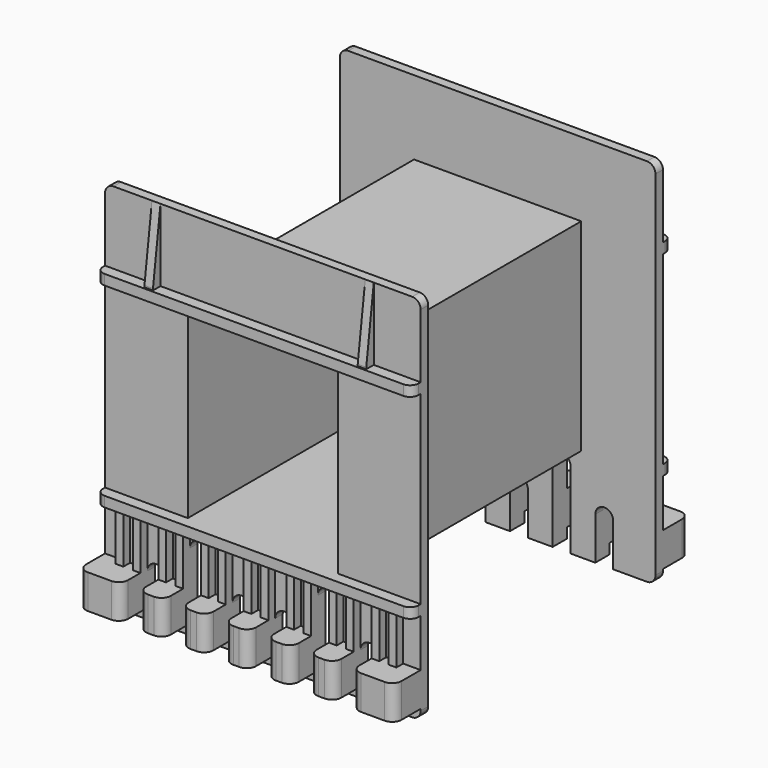
from build123d import *

# Parameters (mm, degrees)
F2_START  = 16.65
F1_W      = 37
F1_H      = 43.4
F1_W_2    = 17.6
F1_H_2    = 21.7
F2_DEPTH  = 1.1
F3_W      = 37
F3_H      = 1.2
F4_DEPTH  = 1.3
F6_DEPTH  = 1.3
F7_W      = 1
F7_H      = 8.5
F9_DEPTH  = 1.1
F8_W      = 1
F8_H      = 8.5
F10_DEPTH = 1.1
F11_SIZE2 = 8.3
F11_SIZE  = 1.1
F12_W     = 0.9
F12_H     = 10.8
F13_DEPTH = 1
F14_W     = 2.05
F14_H     = 4
F14_W_2   = 0.9
F14_W_3   = 1.1
F14_H_2   = 3.9999026618
F15_DEPTH = 3.9
F16_W     = 2.1
F16_H     = 5
F17_W     = 2.1
F17_H     = 9
F18_W     = 2.1
F18_H     = 5
F19_W     = 2.1
F19_H     = 5
F20_W     = 2.1
F20_H     = 9
F21_W     = 2.1
F21_H     = 5
F22_DEPTH = 2.5
F23_R     = 1
F24_R     = 1.1
F27_W     = 19.6
F27_H     = 23.7
F27_W_2   = 17.6
F27_H_2   = 21.7
F28_DEPTH = 17.5
F29_W     = 37.0475144535
F29_H     = 1.2455911213
F30_DEPTH = 2


with BuildPart() as f2:
    # F1 (on face) → F2 (new body)
    with BuildSketch(Plane.XZ.offset(F2_START)):
        with Locations((0, 21.6187323556)):
            Rectangle(F1_W, F1_H)
        with Locations((0, 22.7687323556)):
            Rectangle(F1_W_2, F1_H_2, mode=Mode.SUBTRACT)
    extrude(amount=F2_DEPTH)

    # F3 (on face) → F4 (join)
    with BuildSketch(Plane.XZ.offset(17.75)):
        with Locations((0, 34.2187323556)):
            Rectangle(F3_W, F3_H)
    extrude(amount=F4_DEPTH)

    # F5 (on face) → F6 (join)
    with BuildSketch(Plane.XZ.offset(17.75)):
        Polygon((-18.5, 11.9187323556), (-18.5, 10.7187323556), (18.5, 10.7187323556), (18.5, 11.9187323556), (8.8, 11.9187323556), (-8.8, 11.9187323556), align=None)
    extrude(amount=F6_DEPTH)

    # F7 (on face) → F9 (join)
    with BuildSketch(Plane.XZ.offset(17.75)):
        with Locations((-12.5, 39.0687323556)):
            Rectangle(F7_W, F7_H)
    extrude(amount=F9_DEPTH)

    # F8 (on face) → F10 (join)
    with BuildSketch(Plane.XZ.offset(17.75)):
        with Locations((12.5, 39.0687323556)):
            Rectangle(F8_W, F8_H)
    extrude(amount=F10_DEPTH)

    # F11
    f11_edges = [f2.edges().sort_by_distance(p)[0] for p in [
        (-12.5, -18.85, 43.318732),
        (12.5, -18.85, 43.318732),
    ]]
    f11_side = f2.faces().sort_by_distance((0, -17.25641, 43.318732))[0]
    chamfer(f11_edges, length=F11_SIZE, length2=F11_SIZE2, reference=f11_side)

    # F12 (on face) → F13 (join)
    with BuildSketch(Plane.XZ.offset(17.75)):
        with Locations((-16, 5.3187323556)):
            Rectangle(F12_W, F12_H)
        with Locations((-14, 5.3187323556)):
            Rectangle(F12_W, F12_H)
        with Locations((-11, 5.3187323556)):
            Rectangle(F12_W, F12_H)
        with Locations((-9, 5.3187323556)):
            Rectangle(F12_W, F12_H)
        with Locations((-6, 5.3187323556)):
            Rectangle(F12_W, F12_H)
        with Locations((-4, 5.3187323556)):
            Rectangle(F12_W, F12_H)
        with Locations((-1, 5.3187323556)):
            Rectangle(F12_W, F12_H)
        with Locations((1, 5.3187323556)):
            Rectangle(F12_W, F12_H)
        with Locations((4, 5.3187323556)):
            Rectangle(F12_W, F12_H)
        with Locations((6, 5.3187323556)):
            Rectangle(F12_W, F12_H)
        with Locations((9, 5.3187323556)):
            Rectangle(F12_W, F12_H)
        with Locations((11, 5.3187323556)):
            Rectangle(F12_W, F12_H)
        with Locations((14, 5.3187323556)):
            Rectangle(F12_W, F12_H)
        with Locations((16, 5.3187323556)):
            Rectangle(F12_W, F12_H)
    extrude(amount=F13_DEPTH)

    # F14 (on face) → F15 (join)
    with BuildSketch(Plane.XZ.offset(17.75)):
        with Locations((-17.475, 3.1187323556)):
            Rectangle(F14_W, F14_H)
        with Locations((-16, 3.1187323556)):
            Rectangle(F14_W_2, F14_H)
        with Locations((-15, 3.1187323556)):
            Rectangle(F14_W_3, F14_H)
        with Locations((-14, 3.1187323556)):
            Rectangle(F14_W_2, F14_H)
        with Locations((-11, 3.1186836865)):
            Rectangle(F14_W_2, F14_H_2)
        with Locations((-10, 3.1186836865)):
            Rectangle(F14_W_3, F14_H_2)
        with Locations((-9, 3.1186836865)):
            Rectangle(F14_W_2, F14_H_2)
        with Locations((-6, 3.1186836865)):
            Rectangle(F14_W_2, F14_H_2)
        with Locations((-5, 3.1186836865)):
            Rectangle(F14_W_3, F14_H_2)
        with Locations((-4, 3.1186836865)):
            Rectangle(F14_W_2, F14_H_2)
        with Locations((-1, 3.1187323556)):
            Rectangle(F14_W_2, F14_H)
        with Locations((0, 3.1187323556)):
            Rectangle(F14_W_3, F14_H)
        with Locations((1, 3.1187323556)):
            Rectangle(F14_W_2, F14_H)
        with Locations((4, 3.1187323556)):
            Rectangle(F14_W_2, F14_H)
        with Locations((5, 3.1187323556)):
            Rectangle(F14_W_3, F14_H)
        with Locations((6, 3.1187323556)):
            Rectangle(F14_W_2, F14_H)
        with Locations((9, 3.1187323556)):
            Rectangle(F14_W_2, F14_H)
        with Locations((10, 3.1187323556)):
            Rectangle(F14_W_3, F14_H)
        with Locations((11, 3.1187323556)):
            Rectangle(F14_W_2, F14_H)
        with Locations((14, 3.1187323556)):
            Rectangle(F14_W_2, F14_H)
        with Locations((15, 3.1187323556)):
            Rectangle(F14_W_3, F14_H)
        with Locations((16, 3.1187323556)):
            Rectangle(F14_W_2, F14_H)
        with Locations((17.475, 3.1187323556)):
            Rectangle(F14_W, F14_H)
    extrude(amount=F15_DEPTH)

    # F16 (on face) + F17 (on face) + F18 (on face) + F19 (on face) + F20 (on face) + F21 (on face) → F22 (cut, symmetric)
    with BuildSketch(Plane.XZ.offset(17.75)):
        with Locations((-12.5, 2.4187323556)):
            Rectangle(F16_W, F16_H)
        with BuildLine():
            ThreePointArc((-11.45, 4.9187323556), (-12.5, 5.9687323556), (-13.55, 4.9187323556))
            Line((-13.55, 4.9187323556), (-11.45, 4.9187323556))
        make_face()
    with BuildSketch(Plane.XZ.offset(17.75)):
        with Locations((-7.5, 4.4187323556)):
            Rectangle(F17_W, F17_H)
        with BuildLine():
            ThreePointArc((-6.45, 8.9187323556), (-7.5, 9.9687323556), (-8.55, 8.9187323556))
            Line((-8.55, 8.9187323556), (-6.45, 8.9187323556))
        make_face()
    with BuildSketch(Plane.XZ.offset(17.75)):
        with BuildLine():
            ThreePointArc((-1.45, 4.9187323556), (-2.5, 5.9687323556), (-3.55, 4.9187323556))
            Line((-3.55, 4.9187323556), (-1.45, 4.9187323556))
        make_face()
        with Locations((-2.5, 2.4187323556)):
            Rectangle(F18_W, F18_H)
    with BuildSketch(Plane.XZ.offset(17.75)):
        with BuildLine():
            ThreePointArc((3.55, 4.9187323556), (2.5, 5.9687323556), (1.45, 4.9187323556))
            Line((1.45, 4.9187323556), (3.55, 4.9187323556))
        make_face()
        with Locations((2.5, 2.4187323556)):
            Rectangle(F19_W, F19_H)
    with BuildSketch(Plane.XZ.offset(17.75)):
        with BuildLine():
            ThreePointArc((8.55, 8.9187323556), (7.5, 9.9687323556), (6.45, 8.9187323556))
            Line((6.45, 8.9187323556), (8.55, 8.9187323556))
        make_face()
        with Locations((7.5, 4.4187323556)):
            Rectangle(F20_W, F20_H)
    with BuildSketch(Plane.XZ.offset(17.75)):
        with BuildLine():
            ThreePointArc((13.55, 4.9187323556), (12.5, 5.9687323556), (11.45, 4.9187323556))
            Line((11.45, 4.9187323556), (13.55, 4.9187323556))
        make_face()
        with Locations((12.5, 2.4187323556)):
            Rectangle(F21_W, F21_H)
    extrude(amount=F22_DEPTH, both=True, mode=Mode.SUBTRACT)

    # F23
    f23_edges = [f2.edges().sort_by_distance(p)[0] for p in [
        (-18.5, -17.2, 43.318732),
        (18.5, -17.2, 43.318732),
        (18.5, -17.2, -0.081268),
        (-18.5, -17.2, -0.081268),
        (-18.5, -19.05, 34.218732),
        (18.5, -19.05, 34.218732),
        (18.5, -19.05, 11.318732),
        (-18.5, -19.05, 11.318732),
    ]]
    fillet(f23_edges, radius=F23_R)

    # F24
    f24_edges = [f2.edges().sort_by_distance(p)[0] for p in [
        (-18.5, -21.65, 3.118732),
        (-13.55, -21.65, 3.118732),
        (-11.45, -21.65, 3.118684),
        (-8.55, -21.65, 3.118684),
        (-6.45, -21.65, 3.118684),
        (-3.55, -21.65, 3.118684),
        (-1.45, -21.65, 3.118732),
        (1.45, -21.65, 3.118732),
        (3.55, -21.65, 3.118732),
        (6.45, -21.65, 3.118732),
        (8.55, -21.65, 3.118732),
        (11.45, -21.65, 3.118732),
        (13.55, -21.65, 3.118732),
        (18.5, -21.65, 3.118732),
    ]]
    fillet(f24_edges, radius=F24_R)


with BuildPart() as f25_1:
    # F25: instance of F2
    add(f2.part.mirror(Plane.XZ))


with BuildPart() as f2_1:
    add(f2.part)

    add(f25_1.part)  # F28 merges F25_1
    # F27 (on face) → F28 (join, symmetric)
    with BuildSketch(Plane.XZ):
        with Locations((0, 22.7687323556)):
            Rectangle(F27_W, F27_H)
        with Locations((0, 22.7687323556)):
            Rectangle(F27_W_2, F27_H_2, mode=Mode.SUBTRACT)
    extrude(amount=F28_DEPTH, both=True)

    # F29 (on face) → F30 (cut)
    with BuildSketch(Plane.XZ.offset(17.75)):
        with Locations((-0.0237572268, 0.4959367949)):
            Rectangle(F29_W, F29_H)
    extrude(amount=F30_DEPTH, mode=Mode.SUBTRACT)


solid = f2_1.part
